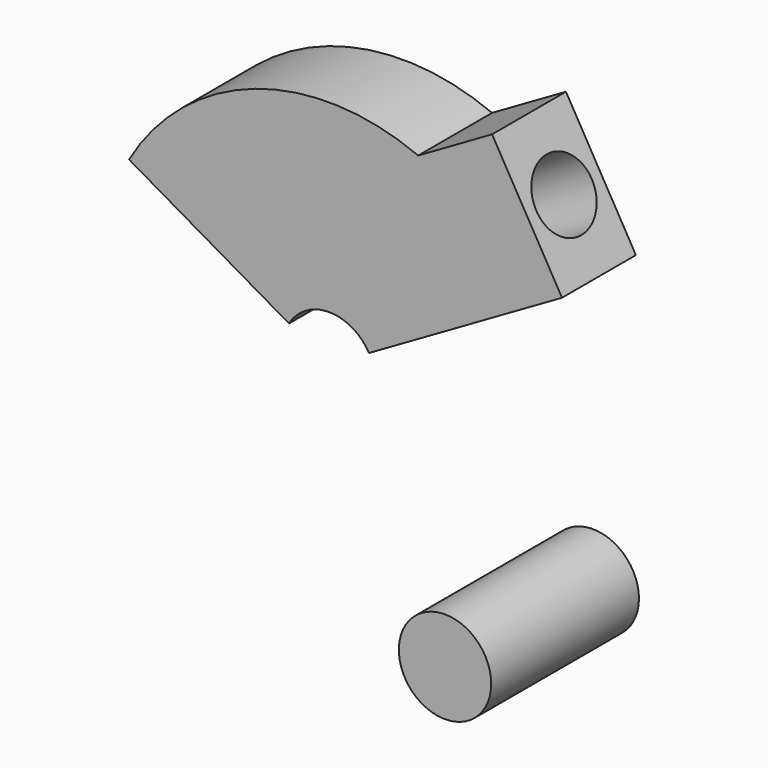
from build123d import *

# Parameters (mm, degrees)
F1_DEPTH = 12.7
F2_R     = 3.175
F3_DEPTH = 50.8
F2_R_2   = 9.525
F4_DEPTH = 25.4
F5_R     = 12.7
F6_DEPTH = 50.8


with BuildPart() as f1:
    # F0 (on Front) → F1 (new body, symmetric)
    with BuildSketch(Plane.XZ):
        with BuildLine():
            ThreePointArc((-10.9985226281, 6.35), (0, 12.7), (10.9985226281, 6.35))
            Line((10.9985226281, 6.35), (54.9926131403, 31.75))
            ThreePointArc((54.9926131403, 31.75), (41.960002336, 47.6613911249), (24.5253888692, 58.5726497677))
            ThreePointArc((24.5253888692, 58.5726497677), (-20.2959743259, 60.1691235283), (-54.9926131403, 31.75))
            Line((-54.9926131403, 31.75), (-10.9985226281, 6.35))
        make_face()
        with BuildLine():
            ThreePointArc((24.5253888692, 58.5726497677), (41.960002336, 47.6613911249), (54.9926131403, 31.75))
            Line((54.9926131403, 31.75), (64.087460216, 37.0009124074))
            Line((64.087460216, 37.0009124074), (44.8561061004, 70.310594834))
            Line((44.8561061004, 70.310594834), (24.5253888692, 58.5726497677))
        make_face()
    extrude(amount=F1_DEPTH, both=True)

    # F2 (on face) → F3 (cut)
    with BuildSketch(Plane(origin=(64.087460216, 0, 37.0009124074), x_dir=(0, 1, 0), z_dir=(0.8660254038, 0, 0.5))):
        with Locations((0, 19.2313541156)):
            Circle(F2_R)
    extrude(amount=-F3_DEPTH, mode=Mode.SUBTRACT)

    # F2 (on face) → F4 (cut)
    with BuildSketch(Plane(origin=(64.087460216, 0, 37.0009124074), x_dir=(0, 1, 0), z_dir=(0.8660254038, 0, 0.5))):
        with Locations((0, 19.2313541156)):
            Circle(F2_R_2)
        with Locations((0, 19.2313541156)):
            Circle(F2_R, mode=Mode.SUBTRACT)
    extrude(amount=-F4_DEPTH, mode=Mode.SUBTRACT)


with BuildPart() as f6:
    # F5 (on Front) → F6 (new body)
    with BuildSketch(Plane.XZ):
        with Locations((62.3870678246, -37.413392216)):
            Circle(F5_R)
    extrude(amount=F6_DEPTH)


solid = Compound([f1.part, f6.part])
